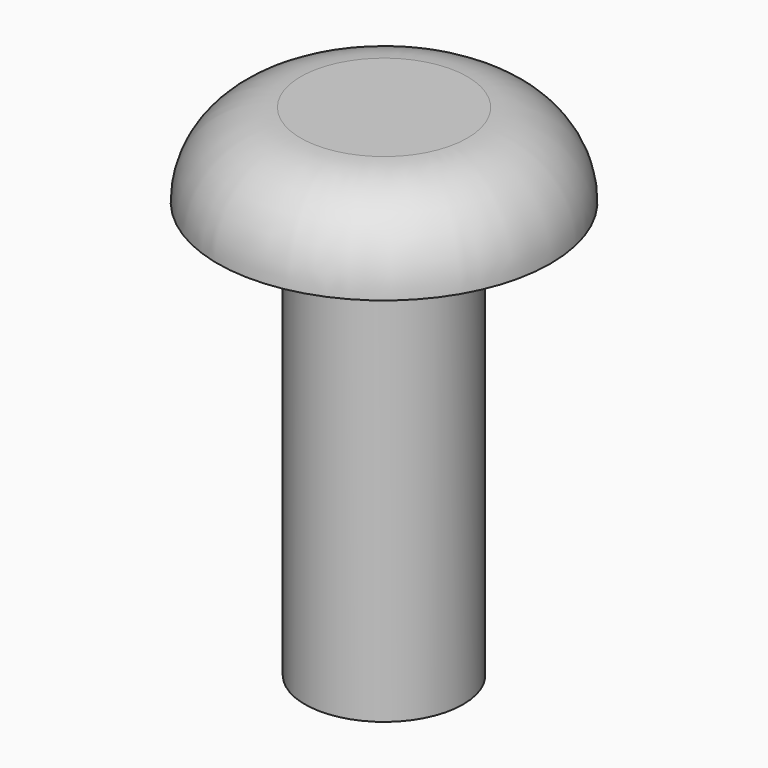
from build123d import *

# Parameters (mm, degrees)
F0_R     = 2.413
F1_DEPTH = 12.7
F2_R     = 5.08
F3_DEPTH = 2.54
F4_R     = 2.53999


# Not quite as in the source:
# - a fillet or chamfer is up to 0.001 mm smaller than in the source, because OpenCascade refuses the exact size


with BuildPart() as f1:
    # F0 (on Top) → F1 (new body)
    with BuildSketch(Plane.XY):
        Circle(F0_R)
    extrude(amount=F1_DEPTH)

    # F2 (on face) → F3 (join)
    with BuildSketch(Plane.XY.offset(12.7)):
        Circle(F2_R)
    extrude(amount=F3_DEPTH)

    # F4 (radius 2.54 in the source; OpenCascade refuses exactly that, so slightly less here)
    f4_edges = [f1.edges().sort_by_distance(p)[0] for p in [
        (-5.08, 0, 15.24),
    ]]
    fillet(f4_edges, radius=F4_R)


solid = f1.part
